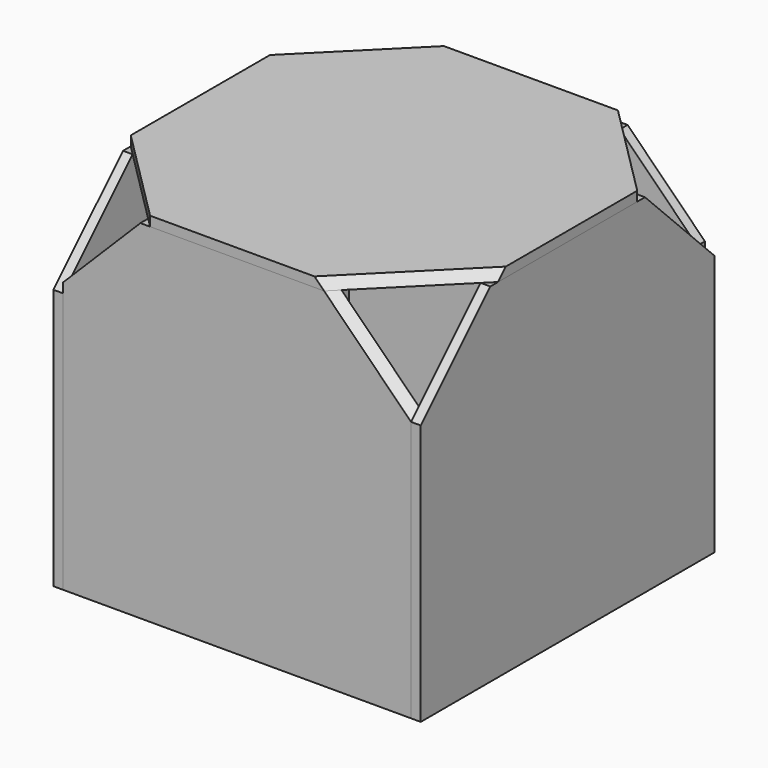
from build123d import *

# Parameters (mm, degrees)
F3_START   = 38.1
F3_DEPTH   = 2.1166666667
F4_START   = -38.1
F4_DEPTH   = 2.1166666667
F5_START   = 38.1
F5_DEPTH   = 2.1166666667
F6_START   = -38.1
F6_DEPTH   = 2.1166666667
F7_START   = 38.1
F7_DEPTH   = 2.1166666667
F9_SIZE2   = 1.496456
F9_SIZE    = 2.116657
F9_2_SIZE2 = 1.496456
F9_2_SIZE  = 2.116657


# Not quite as in the source:
# - a fillet or chamfer is up to 0.001 mm smaller than in the source, because OpenCascade refuses the exact size


with BuildPart() as f3:
    # F0 (on Front) → F3 (new body)
    with BuildSketch(Plane.XZ.offset(F3_START)):
        Polygon((38.1, 21.1666666667), (21.1666666667, 38.1), (-21.1666666667, 38.1), (-38.1, 21.1666666667), (-38.1, -21.1666666667), (-21.1666666667, -38.1), (21.1666666667, -38.1), (38.1, -21.1666666667), align=None)
        Polygon((-21.1666666667, -38.1), (-38.1, -21.1666666667), (-38.1, -38.1), align=None)
        Polygon((38.1, -38.1), (38.1, -21.1666666667), (21.1666666667, -38.1), align=None)
    extrude(amount=F3_DEPTH)

    # F9#2 (size 2.1166666667 and 1.4964661159 in the source; OpenCascade refuses exactly that, so slightly less here)
    f9_2_edges = [f3.edges().sort_by_distance(p)[0] for p in [
        (29.633333, -40.216667, 29.633333),
    ]]
    f9_2_side = f3.faces().sort_by_distance((29.633333, -39.158333, 29.633333))[0]
    chamfer(f9_2_edges, length=F9_2_SIZE, length2=F9_2_SIZE2, reference=f9_2_side)


with BuildPart() as f4:
    # F0 (on Front) → F4 (new body)
    with BuildSketch(Plane.XZ.offset(F4_START)):
        Polygon((38.1, 21.1666666667), (21.1666666667, 38.1), (-21.1666666667, 38.1), (-38.1, 21.1666666667), (-38.1, -21.1666666667), (-21.1666666667, -38.1), (21.1666666667, -38.1), (38.1, -21.1666666667), align=None)
        Polygon((38.1, -38.1), (38.1, -21.1666666667), (21.1666666667, -38.1), align=None)
        Polygon((-21.1666666667, -38.1), (-38.1, -21.1666666667), (-38.1, -38.1), align=None)
    extrude(amount=-F4_DEPTH)


with BuildPart() as f5:
    # F1 (on Right) → F5 (new body)
    with BuildSketch(Plane.YZ.offset(F5_START)):
        Polygon((21.1666666667, 38.1), (-21.1666666667, 38.1), (-40.2166666667, 19.05), (-40.2166666667, -19.05), (-21.1666666667, -38.1), (21.1666666667, -38.1), (40.2166666667, -19.05), (40.2166666667, 19.05), align=None)
        Polygon((-21.1666666667, -38.1), (-40.2166666667, -19.05), (-40.2166666667, -38.1), align=None)
        Polygon((40.2166666667, -38.1), (40.2166666667, -19.05), (21.1666666667, -38.1), align=None)
    extrude(amount=F5_DEPTH)


with BuildPart() as f6:
    # F1 (on Right) → F6 (new body)
    with BuildSketch(Plane.YZ.offset(F6_START)):
        Polygon((21.1666666667, 38.1), (-21.1666666667, 38.1), (-40.2166666667, 19.05), (-40.2166666667, -19.05), (-21.1666666667, -38.1), (21.1666666667, -38.1), (40.2166666667, -19.05), (40.2166666667, 19.05), align=None)
        Polygon((40.2166666667, -38.1), (40.2166666667, -19.05), (21.1666666667, -38.1), align=None)
        Polygon((-21.1666666667, -38.1), (-40.2166666667, -19.05), (-40.2166666667, -38.1), align=None)
    extrude(amount=-F6_DEPTH)


with BuildPart() as f7:
    # F2 (on Top) → F7 (new body)
    with BuildSketch(Plane.XY.offset(F7_START)):
        Polygon((40.2166666667, 19.05), (38.1, 21.1666666667), (38.1, -21.1666666667), (40.2166666667, -19.05), align=None)
        Polygon((-21.1666666667, 38.1), (21.1666666667, 38.1), (19.05, 40.2166666667), (-19.05, 40.2166666667), align=None)
        Polygon((38.1, 21.1666666667), (21.1666666667, 38.1), (-21.1666666667, 38.1), (-38.1, 21.1666666667), (-38.1, -21.1666666667), (-21.1666666667, -38.1), (21.1666666667, -38.1), (38.1, -21.1666666667), align=None)
        Polygon((19.05, -40.2166666667), (21.1666666667, -38.1), (-21.1666666667, -38.1), (-19.05, -40.2166666667), align=None)
        Polygon((-38.1, -21.1666666667), (-38.1, 21.1666666667), (-40.2166666667, 19.05), (-40.2166666667, -19.05), align=None)
    extrude(amount=F7_DEPTH)

    # F9 (size 2.1166666667 and 1.4964661159 in the source; OpenCascade refuses exactly that, so slightly less here)
    f9_edges = [f7.edges().sort_by_distance(p)[0] for p in [
        (29.633333, -29.633333, 40.216667),
    ]]
    f9_side = f7.faces().sort_by_distance((29.633333, -29.633333, 39.158333))[0]
    chamfer(f9_edges, length=F9_SIZE, length2=F9_SIZE2, reference=f9_side)


solid = Compound([f3.part, f4.part, f5.part, f6.part, f7.part])
